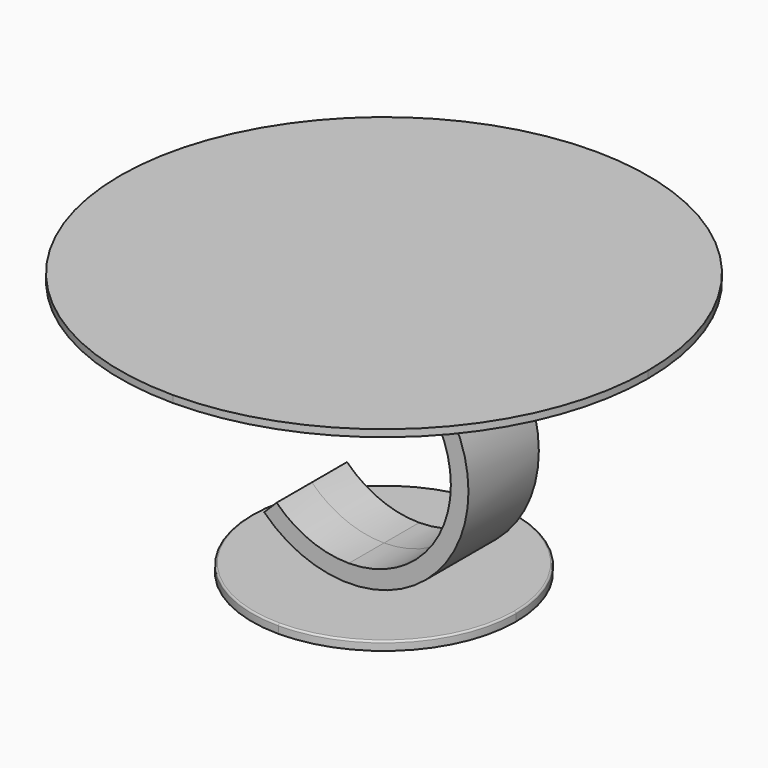
from build123d import *

# Parameters (mm, degrees)
F1_DEPTH      = 300
F1_DEPTH_BACK = 300
F2_DEPTH      = 150
F2_DEPTH_BACK = 150
F3_DEPTH      = 50
F3_DEPTH_BACK = 50
F4_R          = 299.99999
F5_R          = 149.99999
F5_2_R        = 149.99999
F6_R          = 2
F6_2_R        = 2


# Not quite as in the source:
# - a fillet or chamfer is up to 0.001 mm smaller than in the source, because OpenCascade refuses the exact size


with BuildPart() as f1:
    # F0 (on Front) → F1 (new body, two sides)
    with BuildSketch(Plane.XZ) as f1_sk:
        Polygon((-150, 292), (150, 292), (300, 292), (300, 300), (-300, 300), (-300, 292), align=None)
    extrude(amount=F1_DEPTH)
    extrude(f1_sk.sketch, amount=-F1_DEPTH_BACK)

    # F4 (radius 300 in the source; OpenCascade refuses exactly that, so slightly less here)
    f4_edges = [f1.edges().sort_by_distance(p)[0] for p in [
        (-300, 300, 296),
        (-300, -300, 296),
        (300, 300, 296),
        (300, -300, 296),
    ]]
    fillet(f4_edges, radius=F4_R)


with BuildPart() as f2:
    # F0 (on Front) → F2 (new body, two sides)
    with BuildSketch(Plane.XZ) as f2_sk:
        Polygon((-150, 282), (0, 282), (150, 282), (150, 292), (-150, 292), align=None)
    extrude(amount=F2_DEPTH)
    extrude(f2_sk.sketch, amount=-F2_DEPTH_BACK)

    # F5 (radius 150 in the source; OpenCascade refuses exactly that, so slightly less here)
    f5_edges = [f2.edges().sort_by_distance(p)[0] for p in [
        (150, -150, 287),
        (150, 150, 287),
        (-150, 150, 287),
        (-150, -150, 287),
    ]]
    fillet(f5_edges, radius=F5_R)

    # F6
    f6_edges = [f2.edges().sort_by_distance(p)[0] for p in [
        (-150, 0, 282),
        (-106.06602, -106.06602, 282),
        (-106.06602, 106.06602, 282),
        (0, -150, 282),
        (0, 150, 282),
        (106.06602, -106.06602, 282),
        (106.06602, 106.06602, 282),
        (150, 0, 282),
    ]]
    fillet(f6_edges, radius=F6_R)


with BuildPart() as f2b:
    # F0 (on Front) → F2, piece 2 (new body, two sides)
    with BuildSketch(Plane.XZ) as f2_2_sk:
        Polygon((-150, 0), (0, 0), (150, 0), (150, 10), (0, 10), (-150, 10), align=None)
    extrude(amount=F2_DEPTH)
    extrude(f2_2_sk.sketch, amount=-F2_DEPTH_BACK)

    # F5#2 (radius 150 in the source; OpenCascade refuses exactly that, so slightly less here)
    f5_2_edges = [f2b.edges().sort_by_distance(p)[0] for p in [
        (150, -150, 5),
        (150, 150, 5),
        (-150, -150, 5),
        (-150, 150, 5),
    ]]
    fillet(f5_2_edges, radius=F5_2_R)

    # F6#2
    f6_2_edges = [f2b.edges().sort_by_distance(p)[0] for p in [
        (0, -150, 10),
        (-106.06602, -106.06602, 10),
        (106.06602, -106.06602, 10),
        (-150, 0, 10),
        (150, 0, 10),
        (-106.06602, 106.06602, 10),
        (106.06602, 106.06602, 10),
        (0, 150, 10),
    ]]
    fillet(f6_2_edges, radius=F6_2_R)


with BuildPart() as f3:
    # F0 (on Front) → F3 (new body, two sides)
    with BuildSketch(Plane.XZ) as f3_sk:
        with BuildLine():
            Line((0, 30), (0, 10))
            ThreePointArc((0, 10), (136, 146), (0, 282))
            Line((0, 282), (0, 262))
            ThreePointArc((0, 262), (116, 146), (0, 30))
        make_face()
        with BuildLine():
            Line((0, 262), (0, 282))
            ThreePointArc((0, 282), (-52.0449468017, 271.6476164215), (-96.1665222414, 242.1665222414))
            Line((-96.1665222414, 242.1665222414), (-82.0243866176, 228.0243866176))
            ThreePointArc((-82.0243866176, 228.0243866176), (-44.3912781544, 253.1700257713), (0, 262))
        make_face()
        with BuildLine():
            ThreePointArc((-96.1665222414, 49.8334777586), (-52.0449468017, 20.3523835785), (0, 10))
            Line((0, 10), (0, 30))
            ThreePointArc((0, 30), (-44.3912781544, 38.8299742287), (-82.0243866176, 63.9756133824))
            Line((-82.0243866176, 63.9756133824), (-96.1665222414, 49.8334777586))
        make_face()
    extrude(amount=F3_DEPTH)
    extrude(f3_sk.sketch, amount=-F3_DEPTH_BACK)


solid = Compound([f1.part, f2.part, f2b.part, f3.part])
